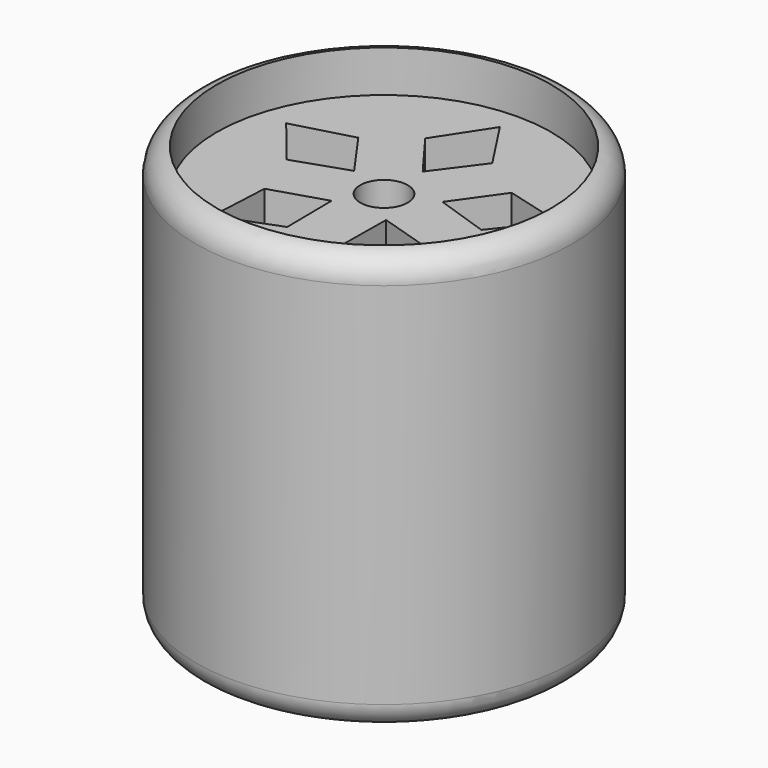
from build123d import *

# Parameters (mm, degrees)
F0_R     = 2
F0_R_2   = 0.284
F1_DEPTH = 2
F0_R_3   = 2.25
F2_DEPTH = 2.5
F4_DEPTH = 12.5


# Not quite as in the source:
# - a fillet or chamfer that OpenCascade refuses, or shapes differently, is made with other operations: its cross-section is extruded or revolved along the edge and cut away or added


with BuildPart() as f1:
    # F0 (on Top) → F1 (new body, symmetric)
    with BuildSketch(Plane.XY):
        Circle(F0_R)
        Circle(F0_R_2, mode=Mode.SUBTRACT)
    extrude(amount=F1_DEPTH, both=True)

    # F0 (on Top) → F2 (join, symmetric)
    with BuildSketch(Plane.XY):
        Circle(F0_R_3)
        Circle(F0_R, mode=Mode.SUBTRACT)
    extrude(amount=F2_DEPTH, both=True)

    # F3 (on Top) → F4 (cut, symmetric)
    with BuildSketch(Plane.XY):
        Polygon((0.4010943762, 1.1171780688), (0, 1.7317327438), (-0.4010943762, 1.1171780688), (0, 0.5784067907), align=None)
        Polygon((-0.8970670571, 0.7371121703), (-1.605488264, 0.5455565888), (-1.1449570143, -0.0258146699), (-0.508610101, 0.1891592692), align=None)
        Polygon((-0.9367568521, -0.6149595416), (-0.9734908601, -1.3479020768), (-0.2877725187, -1.0864742598), (-0.2955828739, -0.4148417807), align=None)
        Polygon((0.3368749389, -1.0705199164), (1.0225932803, -1.3319477334), (0.9858592722, -0.5990051982), (0.344685294, -0.3988874373), align=None)
        Polygon((1.1637124699, 0), (1.6242437196, 0.5713712587), (0.9158225127, 0.7629268403), (0.5273655565, 0.2149739391), align=None)
    extrude(amount=F4_DEPTH, both=True, mode=Mode.SUBTRACT)

    # F5: fillet of radius 0.3 on 3 edges, made by hand

    # F5_s1 → F5_t2 (revolve, cut)
    with BuildSketch(Plane.XZ):
        with BuildLine():
            ThreePointArc((2.25, -2.2041960108), (2.1791287847, -2.3978451782), (2, -2.5))
            Line((2, -2.5), (2.25, -2.5))
            Line((2.25, -2.5), (2.25, -2.2041960108))
        make_face()
    revolve(axis=Axis((0, 0, -2.5), (0, 0, 1)), mode=Mode.SUBTRACT)

    # F5_s3 → F5_t4 (revolve, cut)
    with BuildSketch(Plane.XZ):
        with BuildLine():
            ThreePointArc((2.25, 2.2041960108), (2.1791287847, 2.3978451782), (2, 2.5))
            Line((2, 2.5), (2.25, 2.5))
            Line((2.25, 2.5), (2.25, 2.2041960108))
        make_face()
    revolve(axis=Axis((0, 0, 2.5), (0, 0, 1)), mode=Mode.SUBTRACT)


solid = f1.part
